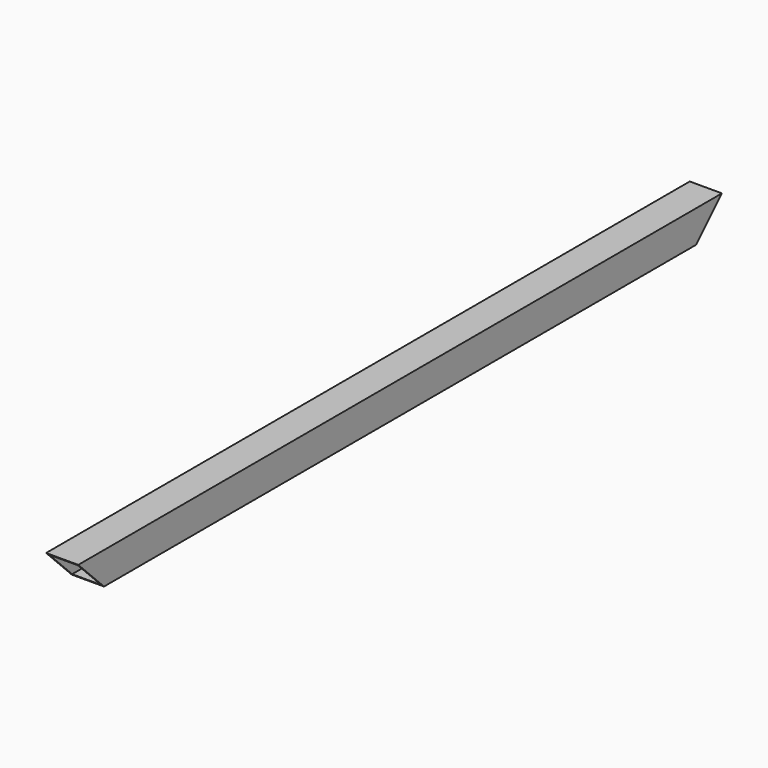
from build123d import *

# Parameters (mm, degrees)
F0_W        = 40
F0_H        = 40
F0_W_2      = 36
F0_H_2      = 36
F1_DEPTH    = 1000
F2_T1_DEPTH = 245.7346390373


# Not quite as in the source:
# - a fillet or chamfer that OpenCascade refuses, or shapes differently, is made with other operations: its cross-section is extruded or revolved along the edge and cut away or added


with BuildPart() as f1:
    # F0 (on Front) → F1 (new body)
    with BuildSketch(Plane.XZ):
        with Locations((20, 20)):
            Rectangle(F0_W, F0_H)
        with Locations((20, 20)):
            Rectangle(F0_W_2, F0_H_2, mode=Mode.SUBTRACT)
    extrude(amount=F1_DEPTH)

    # F2: chamfer of 40 on 2 edges, made by hand

    # F2_s2 → F2_t1 (cut)
    with BuildSketch(Plane.YZ.offset(-102.8673195186)):
        Polygon((-960, 0), (-1000, 40), (-1000, 0), align=None)
        Polygon((-40, 0), (0, 40), (0, 0), align=None)
    extrude(amount=F2_T1_DEPTH, mode=Mode.SUBTRACT)


solid = f1.part
